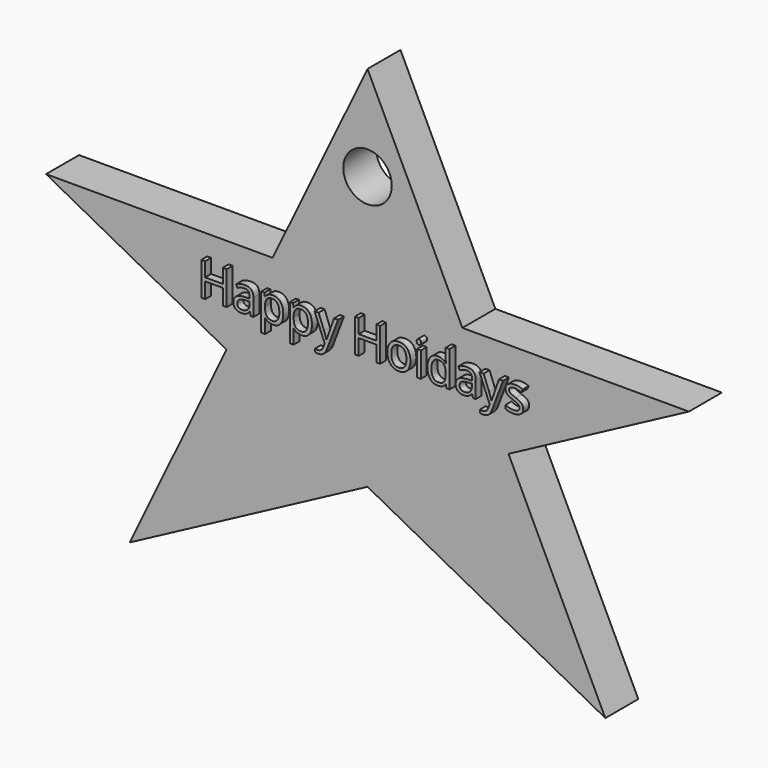
from build123d import *

# Parameters (mm, degrees)
F1_DEPTH     = 12.7
F2_R         = 7.4704924607
F3_DEPTH     = 25.4
F5_TEXT_SIZE = 14.4177383592
F6_DEPTH     = 2.286
F7_TEXT_SIZE = 22.1345092942
F8_DEPTH     = 2.54


# Not quite as in the source:
# - Text() gives the source's letters only with a copy of the font that has no kerning and outlines rounded to 1/6400 em; it was checked with that copy


with BuildPart() as f1:
    # F0 (on Front) → F1 (new body)
    with BuildSketch(Plane.XZ):
        Polygon((-43.4630601364, -11.6461707921), (-73.3147736092, -73.6834090495), (0.0037822486, -34.7349874303), (73.3108944421, -73.6744267555), (43.4641496073, -11.6478890578), (99.0940229482, 17.9039172504), (29.2440229482, 17.9039172504), (0, 78.6778978593), (-29.2438462236, 17.9039172504), (-99.0938462236, 17.9039172504), align=None)
    extrude(amount=F1_DEPTH)

    # F2 (on face) → F3 (cut)
    with BuildSketch(Plane.XZ.offset(12.7)):
        with Locations((0, 49.3930652738)):
            Circle(F2_R)
    extrude(amount=-F3_DEPTH, mode=Mode.SUBTRACT)

    # F5 (on face) → F6 (join)
    with BuildSketch(Plane.XZ.offset(12.7)):
        with Locations((-50.8338462236, 1.4271456318)):
            Text('Happy Hoidays', F5_TEXT_SIZE, font='Open Sans', text_align=(TextAlign.LEFT, TextAlign.BOTTOM))
    extrude(amount=F6_DEPTH)

    # F7 (on face) → F8 (cut)
    with BuildSketch(Plane(origin=(0, 0, 0), x_dir=(-1, 0, 0), z_dir=(0, 1, 0))):
        with Locations((-25.4340229482, -5.448070623)):
            Text('5122', F7_TEXT_SIZE, font='Open Sans', text_align=(TextAlign.LEFT, TextAlign.BOTTOM))
    extrude(amount=-F8_DEPTH, mode=Mode.SUBTRACT)


solid = f1.part
